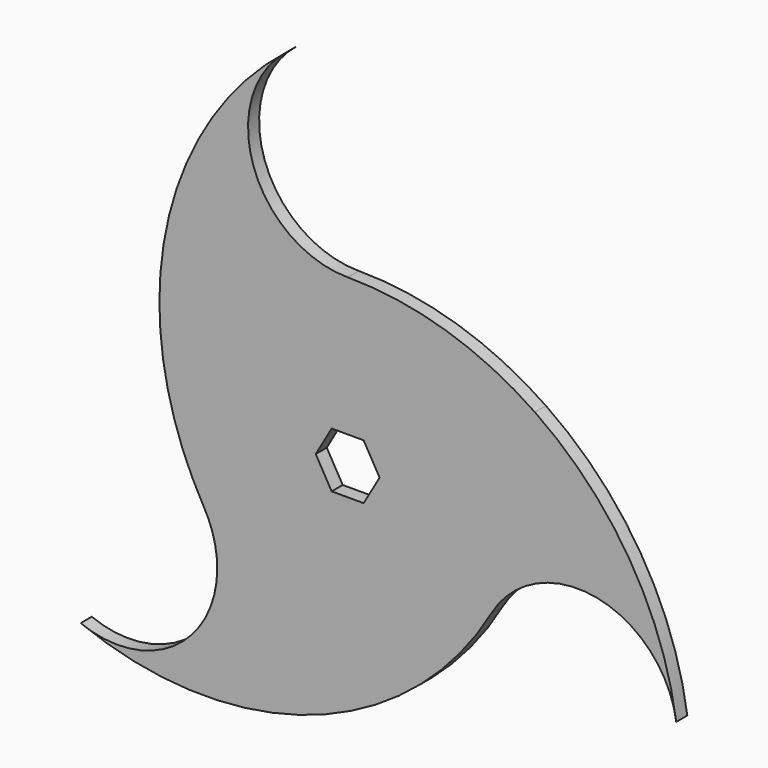
from build123d import *

# Parameters (mm, degrees)
F1_DEPTH = 3.175


with BuildPart() as f1:
    # F0 (on Front) → F1 (new body)
    with BuildSketch(Plane.XZ):
        with BuildLine():
            ThreePointArc((32.9955675162, -19.0500006373), (36.8017738864, -9.8610059738), (38.1, 0))
            ThreePointArc((38.1, 0), (26.9407683703, 26.9407683561), (2.01e-08, 38.1))
            ThreePointArc((2.01e-08, 38.1), (-32.9955680289, 19.0499997494), (-32.9955675847, -19.0500005187))
            ThreePointArc((-32.9955675847, -19.0500005187), (-6.85e-08, -38.1), (32.9955675162, -19.0500006373))
        make_face()
        Polygon((3.6661742094, 6.35), (7.3323484187, 0), (3.6661742094, -6.35), (-3.6661742094, -6.35), (-7.3323484187, 0), (-3.6661742094, 6.35), align=None, mode=Mode.SUBTRACT)
        with BuildLine():
            ThreePointArc((2.01e-08, 38.1), (26.9407683703, 26.9407683561), (38.1, 0))
            ThreePointArc((38.1, 0), (36.8017738864, -9.8610059738), (32.9955675162, -19.0500006373))
            ThreePointArc((32.9955675162, -19.0500006373), (40.6079799838, -0.6720115922), (43.2044321158, 19.05))
            ThreePointArc((43.2044321158, 19.05), (43.1497599719, 21.9360086092), (42.9858219927, 24.8178758988))
            ThreePointArc((42.9858219927, 24.8178758988), (22.4955313049, 34.7037847321), (2.01e-08, 38.1))
        make_face()
        with BuildLine():
            ThreePointArc((-32.9955675847, -19.0500005187), (-32.9955680289, 19.0499997494), (2.01e-08, 38.1))
            ThreePointArc((2.01e-08, 38.1), (-22.4955312856, 34.703784738), (-42.9858219927, 24.8178758988))
            ThreePointArc((-42.9858219927, 24.8178758988), (-41.3021247691, 2.1298089138), (-32.9955675847, -19.0500005187))
        make_face()
        with BuildLine():
            ThreePointArc((-42.9858219927, 24.8178758988), (-22.4955312856, 34.703784738), (2.01e-08, 38.1))
            ThreePointArc((2.01e-08, 38.1), (-21.6006695494, 53.4773083041), (-14.1409580475, 78.92142827))
            ThreePointArc((-14.1409580475, 78.92142827), (-34.2450737922, 54.8987950557), (-42.9858219927, 24.8178758988))
        make_face()
        with BuildLine():
            ThreePointArc((0, -49.6357517976), (18.8065932705, -36.833594191), (32.9955675162, -19.0500006373))
            ThreePointArc((32.9955675162, -19.0500006373), (-6.85e-08, -38.1), (-32.9955675847, -19.0500005187))
            ThreePointArc((-32.9955675847, -19.0500005187), (-18.8065933208, -36.8335941444), (0, -49.6357517976))
        make_face()
        with BuildLine():
            ThreePointArc((43.2044321158, 19.05), (40.6079799838, -0.6720115922), (32.9955675162, -19.0500006373))
            ThreePointArc((32.9955675162, -19.0500006373), (57.1130420252, -8.0319255321), (75.4184408331, -27.2142854025))
            ThreePointArc((75.4184408331, -27.2142854025), (64.6662880971, 2.2077062576), (42.9858219927, 24.8178758988))
            ThreePointArc((42.9858219927, 24.8178758988), (43.1497599719, 21.9360086092), (43.2044321158, 19.05))
        make_face()
        with BuildLine():
            ThreePointArc((0, -49.6357517976), (-18.8065933208, -36.8335941444), (-32.9955675847, -19.0500005187))
            ThreePointArc((-32.9955675847, -19.0500005187), (-30.7118441482, -24.5633969182), (-29.9329086147, -30.48))
            ThreePointArc((-29.9329086147, -30.48), (-39.9745190131, -49.4079816151), (-61.2774832447, -51.7071428447))
            ThreePointArc((-61.2774832447, -51.7071428447), (-30.4212145195, -57.1065013952), (0, -49.6357517976))
        make_face()
    extrude(amount=F1_DEPTH)


solid = f1.part
